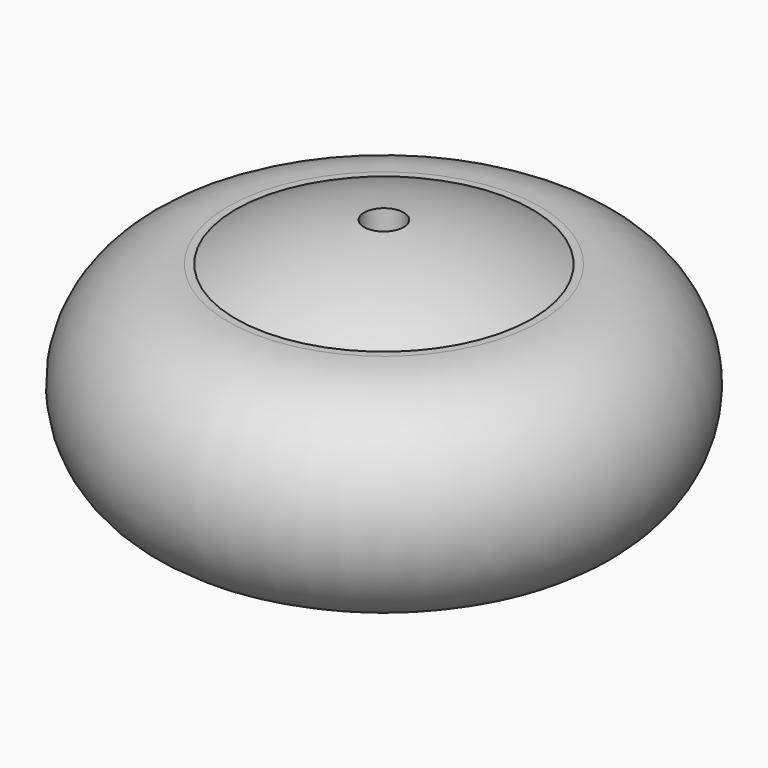
from build123d import *

# Parameters (mm, degrees)
F2_R          = 1.5
F3_DEPTH      = 10.9897371298
F3_DEPTH_BACK = 10.99934016


with BuildPart() as f1:
    # F0 (on Front) → F1 (revolve)
    with BuildSketch(Plane.XZ):
        with BuildLine():
            Line((-11.5125622961, -7.9851364725), (-11.2310720272, -7.9852245345))
            ThreePointArc((-11.2310720272, -7.9852245345), (-5.8128750802, -10.2248932597), (0, -10.9887371298))
            Line((0, -10.9887371298), (0, 10.99834016))
            ThreePointArc((0, 10.99834016), (-5.8099761259, 10.2352713467), (-11.2258712218, 7.997822597))
            Line((-11.2258712218, 7.997822597), (-11.8122072176, 7.9977955632))
            ThreePointArc((-11.8122072176, 7.9977955632), (-19.9927642859, 0.3401750584), (-12.4924337781, -7.9848299277))
            Line((-12.4924337781, -7.9848299277), (-11.5125622961, -7.9851364725))
        make_face()
        with BuildLine():
            ThreePointArc((-12.4924337781, -7.9848299277), (-12.0025027349, -7.9999996085), (-11.5125622961, -7.9851364725))
            Line((-11.5125622961, -7.9851364725), (-12.4924337781, -7.9848299277))
        make_face()
    revolve(axis=Axis((0, 0, 0.0048015151), (0, 0, -1)))

    # F2 (on Top) → F3 (cut, two sides)
    with BuildSketch(Plane.XY) as f3_sk:
        Circle(F2_R)
    extrude(amount=-F3_DEPTH, mode=Mode.SUBTRACT)
    extrude(f3_sk.sketch, amount=F3_DEPTH_BACK, mode=Mode.SUBTRACT)


solid = f1.part
